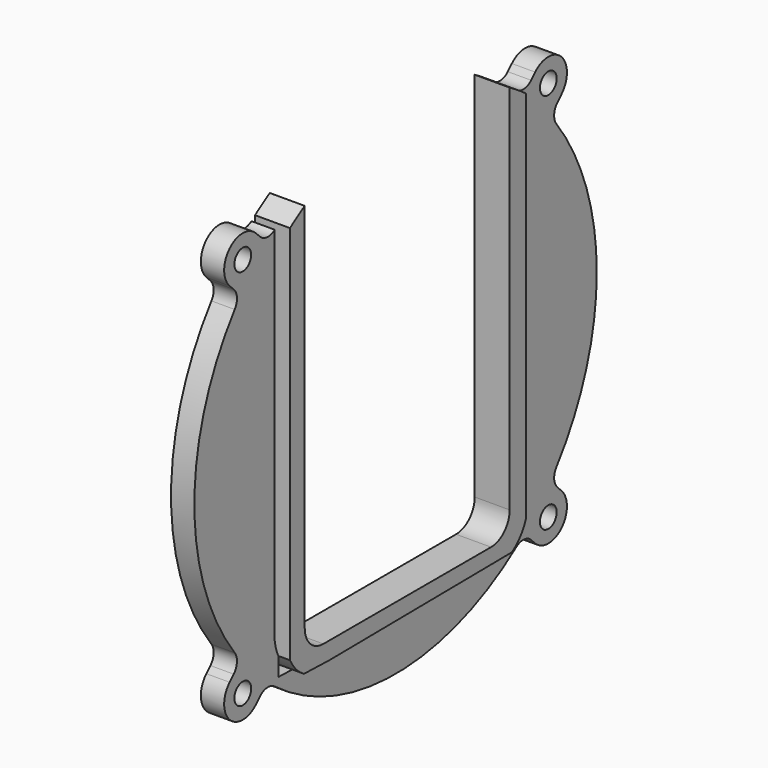
from build123d import *

# Parameters (mm, degrees)
F0_R     = 2.25
F1_DEPTH = 5
F2_DEPTH = 7.5


# Not quite as in the source:
# - a feature of the source that left no trace in its solid (it failed there, or was rolled back) is left out


with BuildPart() as f1:
    # F0 (on Right) → F1 (new body)
    with BuildSketch(Plane.YZ):
        with BuildLine():
            Line((-32.5, -33.3578620553), (-32.5, 43.1248188402))
            ThreePointArc((-32.5, 43.1248188402), (-38.2073481766, 38.1601696185), (-43.1649418054, 32.4466916485))
            ThreePointArc((-43.1649418054, 32.4466916485), (-54, 0), (-43.1649418054, -32.4466916485))
            ThreePointArc((-43.1649418054, -32.4466916485), (-38.1837661841, -38.1837661841), (-32.4466916485, -43.1649418054))
            ThreePointArc((-32.4466916485, -43.1649418054), (0, -54), (32.4466916485, -43.1649418054))
            ThreePointArc((32.4466916485, -43.1649418054), (38.1837661841, -38.1837661841), (43.1649418054, -32.4466916485))
            ThreePointArc((43.1649418054, -32.4466916485), (51.2196586161, -17.1039928453), (54, 0))
            ThreePointArc((54, 0), (51.2196586161, 17.1039928453), (43.1649418054, 32.4466916485))
            ThreePointArc((43.1649418054, 32.4466916485), (38.2073481766, 38.1601696185), (32.5, 43.1248188402))
            Line((32.5, 43.1248188402), (32.5, -33.3578620553))
            ThreePointArc((32.5, -33.3578620553), (32.3474874667, -35.0976869294), (31.8946018815, -36.7844427837))
            Line((31.8946018815, -36.7844427837), (31.8946018815, -41.5552656251))
            Line((31.8946018815, -41.5552656251), (28.1724253923, -41.593369943))
            ThreePointArc((28.1724253923, -41.593369943), (25.4702627091, -42.9065551302), (22.5, -43.3578620553))
            Line((22.5, -43.3578620553), (-22.5, -43.3578620553))
            ThreePointArc((-22.5, -43.3578620553), (-25.2056219122, -42.9848870406), (-27.70941795, -41.8937840689))
            Line((-27.70941795, -41.8937840689), (-31.4624607563, -41.7840279114))
            Line((-31.4624607563, -41.7840279114), (-31.4624607563, -37.7934338552))
            ThreePointArc((-31.4624607563, -37.7934338552), (-32.2371609713, -35.6355135252), (-32.5, -33.3578620553))
        make_face()
        with BuildLine():
            ThreePointArc((-32.5, 43.1248188402), (-32.4733520211, 43.1448885561), (-32.4466916485, 43.1649418054))
            ThreePointArc((-32.4466916485, 43.1649418054), (-34.4603348429, 42.5704269643), (-36.3706059725, 43.4416737844))
            Line((-36.3706059725, 43.4416737844), (-37.4644660941, 44.5355339059))
            ThreePointArc((-37.4644660941, 44.5355339059), (-44.5355339059, 44.5355339059), (-44.5355339059, 37.4644660941))
            Line((-44.5355339059, 37.4644660941), (-43.4416737844, 36.3706059725))
            ThreePointArc((-43.4416737844, 36.3706059725), (-42.5704269643, 34.4603348429), (-43.1649418054, 32.4466916485))
            ThreePointArc((-43.1649418054, 32.4466916485), (-38.2073481766, 38.1601696185), (-32.5, 43.1248188402))
        make_face()
        with Locations((-41, 41)):
            Circle(F0_R, mode=Mode.SUBTRACT)
        with BuildLine():
            ThreePointArc((32.5, 43.1248188402), (38.2073481766, 38.1601696185), (43.1649418054, 32.4466916485))
            ThreePointArc((43.1649418054, 32.4466916485), (42.5704269643, 34.4603348429), (43.4416737844, 36.3706059725))
            Line((43.4416737844, 36.3706059725), (44.5355339059, 37.4644660941))
            ThreePointArc((44.5355339059, 37.4644660941), (44.5355339059, 44.5355339059), (37.4644660941, 44.5355339059))
            Line((37.4644660941, 44.5355339059), (36.3706059725, 43.4416737844))
            ThreePointArc((36.3706059725, 43.4416737844), (34.4603348429, 42.5704269643), (32.4466916485, 43.1649418054))
            ThreePointArc((32.4466916485, 43.1649418054), (32.4733520211, 43.1448885561), (32.5, 43.1248188402))
        make_face()
        with Locations((41, 41)):
            Circle(F0_R, mode=Mode.SUBTRACT)
        with BuildLine():
            ThreePointArc((43.1649418054, -32.4466916485), (38.1837661841, -38.1837661841), (32.4466916485, -43.1649418054))
            ThreePointArc((32.4466916485, -43.1649418054), (34.4603348429, -42.5704269643), (36.3706059725, -43.4416737844))
            Line((36.3706059725, -43.4416737844), (37.4644660941, -44.5355339059))
            ThreePointArc((37.4644660941, -44.5355339059), (44.5355339059, -44.5355339059), (44.5355339059, -37.4644660941))
            Line((44.5355339059, -37.4644660941), (43.4416737844, -36.3706059725))
            ThreePointArc((43.4416737844, -36.3706059725), (42.5704269643, -34.4603348429), (43.1649418054, -32.4466916485))
        make_face()
        with Locations((41, -41)):
            Circle(F0_R, mode=Mode.SUBTRACT)
        with BuildLine():
            ThreePointArc((-32.4466916485, -43.1649418054), (-38.1837661841, -38.1837661841), (-43.1649418054, -32.4466916485))
            ThreePointArc((-43.1649418054, -32.4466916485), (-42.5704269643, -34.4603348429), (-43.4416737844, -36.3706059725))
            Line((-43.4416737844, -36.3706059725), (-44.5355339059, -37.4644660941))
            ThreePointArc((-44.5355339059, -37.4644660941), (-44.5355339059, -44.5355339059), (-37.4644660941, -44.5355339059))
            Line((-37.4644660941, -44.5355339059), (-36.3706059725, -43.4416737844))
            ThreePointArc((-36.3706059725, -43.4416737844), (-34.4603348429, -42.5704269643), (-32.4466916485, -43.1649418054))
        make_face()
        with Locations((-41, -41)):
            Circle(F0_R, mode=Mode.SUBTRACT)
    extrude(amount=F1_DEPTH)


with BuildPart() as f2:
    # F0 (on Right) → F2 (new body)
    with BuildSketch(Plane.YZ):
        with BuildLine():
            ThreePointArc((-27.5, 46.4731105049), (-29.5095624616, 45.2237296486), (-31.4624607563, 43.8875103322))
            Line((-31.4624607563, 43.8875103322), (-31.4624607563, -33.3578620553))
            Line((-31.4624607563, -33.3578620553), (-31.4624607563, -37.7934338552))
            ThreePointArc((-31.4624607563, -37.7934338552), (-29.876567934, -40.1096207532), (-27.70941795, -41.8937840689))
            Line((-27.70941795, -41.8937840689), (-20.8289045841, -42.0950017869))
            Line((-20.8289045841, -42.0950017869), (28.1724253923, -41.593369943))
            ThreePointArc((28.1724253923, -41.593369943), (30.407924685, -39.4787057207), (31.8946018815, -36.7844427837))
            Line((31.8946018815, -36.7844427837), (31.8946018815, -33.3578620553))
            Line((31.8946018815, -33.3578620553), (31.8946018815, 43.5744692546))
            ThreePointArc((31.8946018815, 43.5744692546), (29.7326455843, 45.0773755509), (27.5, 46.4731105049))
            Line((27.5, 46.4731105049), (27.5, -33.3578620553))
            ThreePointArc((27.5, -33.3578620553), (26.0355339059, -36.8933959612), (22.5, -38.3578620553))
            Line((22.5, -38.3578620553), (-22.5, -38.3578620553))
            ThreePointArc((-22.5, -38.3578620553), (-26.0355339059, -36.8933959612), (-27.5, -33.3578620553))
            Line((-27.5, -33.3578620553), (-27.5, 46.4731105049))
        make_face()
    extrude(amount=F2_DEPTH)


solid = Compound([f1.part, f2.part])
